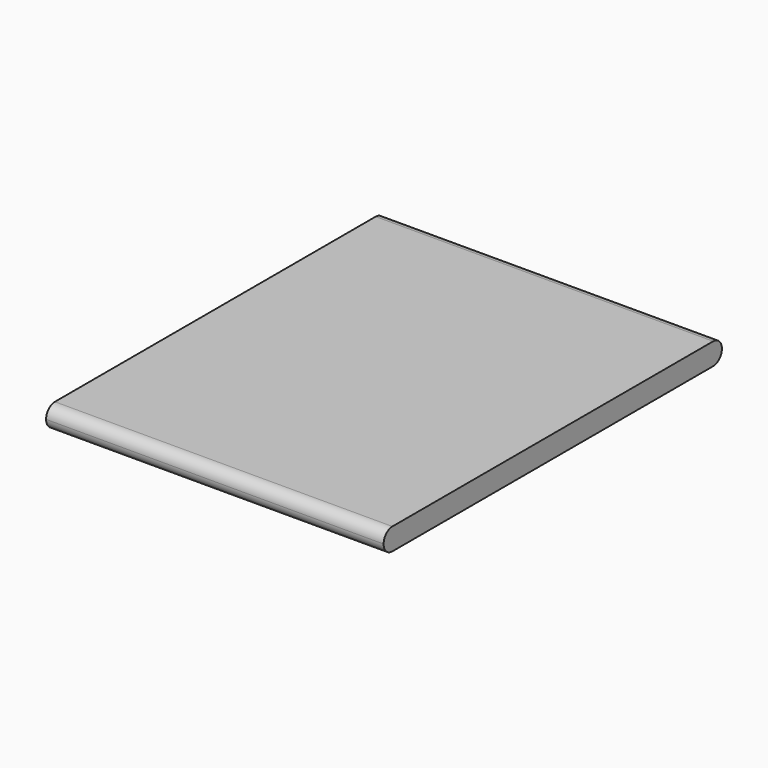
from build123d import *

# Parameters (mm, degrees)
F0_W     = 540
F0_H     = 28
F1_DEPTH = 431
F2_R     = 13.99999


# Not quite as in the source:
# - a fillet or chamfer is up to 0.001 mm smaller than in the source, because OpenCascade refuses the exact size


with BuildPart() as f1:
    # F0 (on Right) → F1 (new body)
    with BuildSketch(Plane.YZ):
        Rectangle(F0_W, F0_H)
    extrude(amount=F1_DEPTH)

    # F2 (radius 14 in the source; OpenCascade refuses exactly that, so slightly less here)
    f2_edges = [f1.edges().sort_by_distance(p)[0] for p in [
        (215.5, 270, 14),
        (215.5, 270, -14),
        (215.5, -270, 14),
        (215.5, -270, -14),
    ]]
    fillet(f2_edges, radius=F2_R)


solid = f1.part
